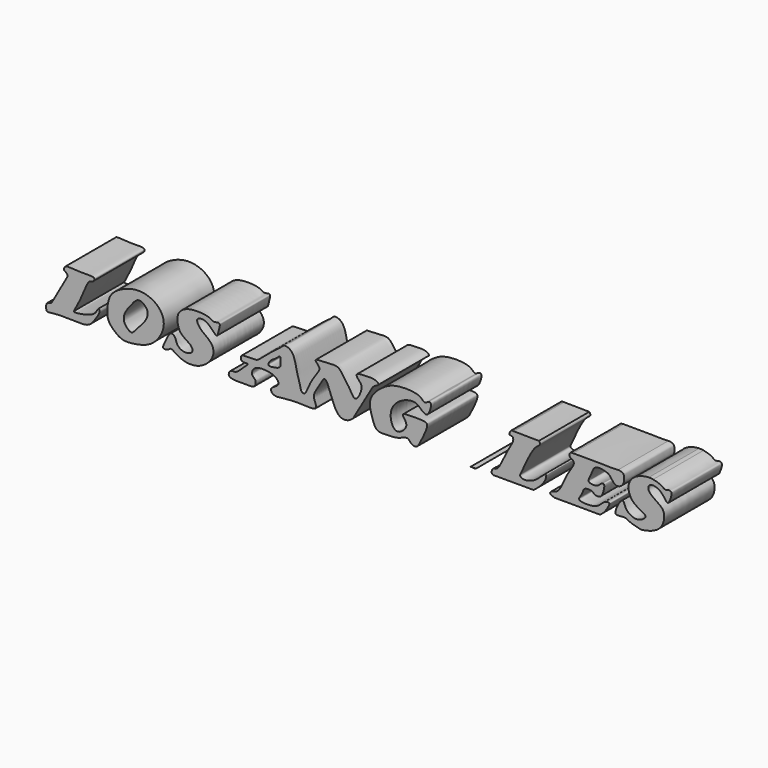
from build123d import *

# Parameters (mm, degrees)
F1_DEPTH = 6.35


# Not quite as in the source:
# - ends of sketch curves that miss each other by under 0.0002 mm in the source are joined


with BuildPart() as f1:
    # F0 (on Front) → F1 (new body)
    with BuildSketch(Plane.XZ):
        with BuildLine():
            add(Edge.make_bspline(
                [(34.4768658758, 14.4737295806), (34.5112801396, 14.4727928271), (34.5458290764, 14.4718709509), (34.5805155984, 14.4709650204)],
                knots=[0.1339558737, 0.1339558737, 0.1339558737, 0.1339558737, 0.1355001097, 0.1355001097, 0.1355001097, 0.1355001097], degree=3))
            add(Edge.make_bspline(
                [(32.5323011747, 9.9067027403), (32.4541670227, 9.9458683585), (32.2751985665, 10.0359966209), (32.4559030704, 10.5729919592), (33.0380168387, 10.4343131271), (33.7711108369, 12.3849964852), (34.5440521378, 13.3995929427), (34.5514155398, 14.0179867081), (34.0324043055, 13.9529814102), (34.2602520135, 14.4479078637), (34.3605137665, 14.4750049981), (34.4768658758, 14.4737295806)],
                knots=[0, 0, 0, 0, 0.027275365, 0.0627849405, 0.0982497275, 0.1752234358, 0.2407914191, 0.2763534131, 0.3071745918, 0.3406755244, 0.3657990569, 0.3657990569, 0.3657990569, 0.3657990569], degree=3))
            add(Edge.make_bspline(
                [(36.5833330066, 9.9053008405), (35.8773893638, 9.9053517321), (34.5279863227, 9.9056091902), (33.1766399411, 9.906295485), (32.5323011747, 9.9067027403)],
                knots=[0.3335392416, 0.3335392416, 0.3335392416, 0.3335392416, 0.4992416228, 0.6501179017, 0.6501179017, 0.6501179017, 0.6501179017], degree=3))
            add(Edge.make_bspline(
                [(37.1199468026, 14.44261028), (37.1519343343, 14.416070329), (37.3677863804, 14.1054250224), (36.4958158296, 13.8301801861), (35.3957687547, 11.0844620344), (35.1546346981, 10.7403969365), (35.5033492144, 10.4136849439), (36.7420555717, 10.676933918), (37.4847481052, 11.5347630695), (37.9200843344, 11.7919258834), (37.7947972791, 11.0937092918), (37.2140296799, 10.4098376288), (36.7884678122, 10.0690914927), (36.5833330066, 9.9053008405)],
                knots=[0.4725030515, 0.4725030515, 0.4725030515, 0.4725030515, 0.5005206768, 0.547700524, 0.6430035296, 0.6760154724, 0.7072056983, 0.7676589039, 0.8284944996, 0.8577824993, 0.8962629012, 0.950243921, 1, 1, 1, 1], degree=3))
            add(Edge.make_bspline(
                [(37.063521727, 14.4425428083), (37.0823137295, 14.442561699), (37.1011223418, 14.4425842176), (37.1199468026, 14.44261028)],
                knots=[0.1692239715, 0.1692239715, 0.1692239715, 0.1692239715, 0.1699378637, 0.1699378637, 0.1699378637, 0.1699378637], degree=3))
            add(Edge.make_bspline(
                [(34.5805155984, 14.4709650204), (35.1314661418, 14.453172138), (36.817595789, 14.4071514338), (37.063521727, 14.4425428083)],
                knots=[0.3721506797, 0.3721506797, 0.3721506797, 0.3721506797, 0.459357375, 0.459357375, 0.459357375, 0.459357375], degree=3))
        make_face()
    extrude(amount=F1_DEPTH)


with BuildPart() as f1b:
    # F0 (on Front) → F1, piece 2 (new body)
    with BuildSketch(Plane.XZ):
        with BuildLine():
            add(Edge.make_bspline(
                [(30.7684035639, 9.9080042533), (30.5910978256, 9.9081525219), (30.4137778692, 9.9083056652), (30.2364464497, 9.9084633249)],
                knots=[0.7877417533, 0.7877417533, 0.7877417533, 0.7877417533, 0.8292299046, 0.8292299046, 0.8292299046, 0.8292299046], degree=3))
            add(Edge.make_bspline(
                [(30.2364464497, 9.9084633249), (30.2480434796, 9.9076282603), (30.4475423088, 9.8919898642), (30.645100962, 9.8532213871), (30.7667153143, 9.907231483), (30.7684035639, 9.9080042533)],
                knots=[0.026563246, 0.026563246, 0.026563246, 0.026563246, 0.0277484383, 0.0470040149, 0.0472770858, 0.0472770858, 0.0472770858, 0.0472770858], degree=3))
        make_face()
    extrude(amount=F1_DEPTH)


with BuildPart() as f1c:
    # F0 (on Front) → F1, piece 3 (new body)
    with BuildSketch(Plane.XZ):
        with BuildLine():
            add(Edge.make_bspline(
                [(38.718625811, 9.9052852467), (38.5135813539, 9.965903255), (38.1634283773, 10.0694614859), (38.3624359939, 10.4577232253), (39.1171957291, 10.4145474294), (39.6140354439, 11.7570882036), (40.264894038, 12.9054629976), (40.6644877345, 13.432394025), (40.6342538489, 13.8855215631), (40.0886665403, 14.024998654), (40.2583159891, 14.4507891646), (40.3653461826, 14.4606033405), (40.5612274768, 14.467808711)],
                knots=[0, 0, 0, 0, 0.0234493646, 0.0400679945, 0.0658311953, 0.1038715824, 0.1427742296, 0.1688455969, 0.1884932671, 0.2104317591, 0.2283583247, 0.2468497136, 0.2468497136, 0.2468497136, 0.2468497136], degree=3))
            add(Edge.make_bspline(
                [(40.8433932409, 9.9057387335), (40.1351970665, 9.905587584), (39.4270009049, 9.9054527643), (38.718625811, 9.9052852467)],
                knots=[0, 0, 0, 0, 0.1663998621, 0.1663998621, 0.1663998621, 0.1663998621], degree=3))
            add(Edge.make_bspline(
                [(43.2678567779, 9.8901794928), (42.4617746641, 9.9157399972), (41.6392296575, 9.9329845193), (40.8433932409, 9.9057387335)],
                knots=[0.8753656822, 0.8753656822, 0.8753656822, 0.8753656822, 0.9071716793, 0.9071716793, 0.9071716793, 0.9071716793], degree=3))
            add(Edge.make_bspline(
                [(45.1012092872, 14.4622358719), (45.4844363537, 14.4274675017), (45.7750792463, 14.3040325549), (45.7165046627, 13.1471962694), (44.7314215276, 12.8484351058), (44.3446618894, 13.7318670905), (43.779898461, 13.9552776294), (42.6721876007, 14.143056728), (42.4200388298, 13.1817012223), (42.1375735513, 12.7160040765), (42.0934433991, 12.3265459652), (43.0723981196, 12.2605262747), (43.3340512659, 12.7193371486), (43.7764141603, 12.8149416944), (43.662126014, 12.1247922037), (43.4210997106, 11.3922556923), (42.6914128218, 11.455909825), (42.5215425357, 11.7876309832), (41.5794702071, 11.8011837957), (41.5631473809, 11.1619219007), (40.9386497254, 10.5104977654), (41.7920834613, 10.3487349178), (43.0985475186, 10.4282046124), (43.5927155966, 11.1933341463), (44.3976497916, 11.3538748898), (43.9912126895, 10.6478167398), (43.6448087091, 10.1523723502), (43.3841416805, 9.9713765802), (43.2678567779, 9.8901794928)],
                knots=[0.3170026618, 0.3170026618, 0.3170026618, 0.3170026618, 0.3434489893, 0.3749791608, 0.4034215732, 0.4328717168, 0.4589348824, 0.4907763547, 0.5210849698, 0.5459241096, 0.5625973731, 0.5919434389, 0.6158108763, 0.6328153746, 0.657443103, 0.6857445259, 0.7103256391, 0.729915535, 0.7580183435, 0.7829258001, 0.809539198, 0.8345757029, 0.8722584856, 0.9036550327, 0.926657814, 0.9511783368, 0.9782105166, 1, 1, 1, 1], degree=3))
            add(Edge.make_bspline(
                [(40.5612274768, 14.467808711), (41.4373321776, 14.4749541476), (43.4065275967, 14.4832914551), (44.404762779, 14.4102661712), (45.1012092872, 14.4622358719)],
                knots=[0.213383647, 0.213383647, 0.213383647, 0.213383647, 0.2482603597, 0.2988779642, 0.2988779642, 0.2988779642, 0.2988779642], degree=3))
        make_face()
    extrude(amount=F1_DEPTH)


with BuildPart() as f1d:
    # F0 (on Front) → F1, piece 4 (new body)
    with BuildSketch(Plane.XZ):
        with BuildLine():
            add(Edge.make_bspline(
                [(48.2063107618, 14.8080410421), (48.361353415, 14.8025450615), (48.5065364369, 14.7871576478), (48.6413690998, 14.7643067953)],
                knots=[0.366400242, 0.366400242, 0.366400242, 0.366400242, 0.3777635297, 0.3777635297, 0.3777635297, 0.3777635297], degree=3))
            add(Edge.make_bspline(
                [(47.4133412883, 9.9057387335), (46.9725338397, 10.0134268872), (46.2515458614, 10.1895948628), (45.850088848, 10.5125088591), (45.138855998, 10.383096561), (44.6552953768, 10.4479064453), (45.2207468206, 11.7372843188), (45.6917339954, 11.9887531473), (45.7921261937, 11.2608218345), (46.5757989122, 10.6369990891), (47.3861596047, 10.7140682616), (48.0851201046, 11.2394276569), (47.3483966756, 11.6465310313), (46.4460471609, 12.0954145822), (45.9472697626, 13.4041358945), (46.7122823199, 14.561768142), (47.8559378649, 14.7943353068), (48.2063107193, 14.8080410436)],
                knots=[0, 0, 0, 0, 0.077437218, 0.1266613719, 0.1855901369, 0.2238421303, 0.3027768951, 0.345087592, 0.3979643199, 0.4667316111, 0.5304178838, 0.5855747405, 0.6398989755, 0.7123026851, 0.7903598777, 0.8691903302, 0.9533376764, 0.9533376764, 0.9533376764, 0.9533376764], degree=3))
            add(Edge.make_bspline(
                [(48.6413690998, 14.7643067953), (49.001027409, 14.7033534715), (49.5110446895, 14.4999664824), (49.8485973579, 14.1905299076), (50.1520312715, 14.3484072118), (50.6416228519, 14.3040310738), (50.3264757069, 13.4051786644), (50.0922791452, 12.9863703016), (49.6665779866, 13.6956729791), (49.1647749556, 14.1531007966), (48.2986025006, 14.3401157398), (47.9873927024, 13.6104758419), (49.0101373653, 12.9095010149), (49.8719114445, 12.3722330399), (49.6878282098, 10.5866768403), (48.4221076097, 10.0353934607), (47.4133412883, 9.9057387335)],
                knots=[0.3777635297, 0.3777635297, 0.3777635297, 0.3777635297, 0.4080744409, 0.4318138392, 0.4518618025, 0.472205762, 0.5054119396, 0.5260348343, 0.5547091476, 0.5863153403, 0.6174273922, 0.6432110306, 0.6815114437, 0.7172127576, 0.7596173353, 0.8144781544, 0.8144781544, 0.8144781544, 0.8144781544], degree=3))
        make_face()
    extrude(amount=F1_DEPTH)


with BuildPart() as f1e:
    # F0 (on Front) → F1, piece 5 (new body)
    with BuildSketch(Plane.XZ):
        with BuildLine():
            add(Edge.make_bspline(
                [(-9.7831104874, 10.7108312697), (-9.5950454946, 11.093317591), (-9.2860023376, 11.7217945983), (-9.0581878575, 12.0865172653), (-8.5637830889, 13.3512127314), (-8.2448274482, 13.9212845659), (-7.8305533182, 13.9063295694), (-7.6446188222, 14.3012483336), (-8.0264709842, 14.4262921763), (-8.8381735222, 14.3667908405), (-10.1439046456, 14.4448887029), (-10.6660898244, 14.4953689384), (-10.8636029298, 14.0294127442), (-10.5848318503, 13.9224699449), (-10.3791844836, 13.6672874639), (-10.4643739569, 13.5103759365), (-10.5048306286, 13.4358583018)],
                knots=[0.0001566694, 0.0001566694, 0.0001566694, 0.0001566694, 0.1031082956, 0.1694222377, 0.2827346198, 0.359654875, 0.417114896, 0.4710627289, 0.5224264412, 0.6128031166, 0.7262449494, 0.793312149, 0.8512485611, 0.8997805232, 0.9524055698, 1, 1, 1, 1], degree=3))
            add(Edge.make_bspline(
                [(-10.5048306286, 13.4358583018), (-11.111802213, 12.355849674), (-11.9073362504, 10.9403243905), (-12.0884096109, 10.6229939383), (-12.5134287105, 10.6403297729), (-12.6107940514, 10.2661819977), (-12.5751779421, 9.6841727582), (-11.8093591696, 9.9133287705), (-9.4218227173, 9.8703548386), (-8.8075229584, 9.8202820579), (-8.0408529888, 10.0242220176), (-7.5418327302, 10.8534472885), (-7.099782311, 11.474480533), (-7.3315011816, 11.8740905081), (-7.5528421638, 11.1609376867), (-8.3507527089, 10.8513853859), (-9.1455907434, 10.6458267455), (-9.7541621378, 10.6050908929), (-9.7812796189, 10.6909704053), (-9.7831104874, 10.7108312697)],
                knots=[0, 0, 0, 0, 0.1223676782, 0.1603825543, 0.201389393, 0.2434286791, 0.2904717262, 0.3475918385, 0.4588206991, 0.5171187103, 0.5761489951, 0.6470845322, 0.7084840664, 0.7415904522, 0.7929674686, 0.8591802712, 0.9271226938, 0.9792659839, 0.9934126503, 0.9934126503, 0.9934126503, 0.9934126503], degree=3))
        make_face()
    extrude(amount=F1_DEPTH)


with BuildPart() as f1f:
    # F0 (on Front) → F1, piece 6 (new body)
    with BuildSketch(Plane.XZ):
        with BuildLine():
            add(Edge.make_bspline(
                [(-5.9119630605, 10.4841180146), (-6.1036939558, 10.6784201151), (-6.4221233493, 11.0480734957), (-6.4396892173, 12.2965647029), (-6.1372585796, 13.5029134325), (-4.8744149654, 14.3512139958), (-3.2895880396, 14.7940159404), (-1.6139891323, 14.3540043474), (-0.6206388277, 13.1356209217), (-0.7539352118, 11.6498263262), (-1.9305291345, 10.1347618448), (-3.6588662383, 9.7564012308), (-5.0124344733, 9.6391651222), (-5.6728543676, 10.241802757), (-5.9119630605, 10.4841180146)],
                knots=[0, 0, 0, 0, 0.060955485, 0.1382878927, 0.2165469674, 0.3017686672, 0.3928667622, 0.484409508, 0.569462374, 0.6528699079, 0.7486580595, 0.8426240387, 0.923982067, 1, 1, 1, 1], degree=3))
        make_face()
        with BuildLine():
            add(Edge.make_bspline(
                [(-4.7054300085, 11.4048924297), (-4.8221480388, 11.7486095831), (-4.5870889049, 12.4341394937), (-4.034172335, 13.1202884214), (-3.4565337255, 13.8525328756), (-2.8552184683, 13.799515972), (-2.1060569123, 13.0199090142), (-2.7246014826, 11.8831877525), (-3.5814458227, 11.0918676538), (-3.9864616129, 10.481888247), (-4.5895573421, 11.0636647467), (-4.7054300085, 11.4048924297)],
                knots=[0, 0, 0, 0, 0.1182200316, 0.2324666919, 0.3420396722, 0.4265101549, 0.5379656341, 0.6653597964, 0.7970240743, 0.882636211, 1, 1, 1, 1], degree=3))
        make_face(mode=Mode.SUBTRACT)
    extrude(amount=F1_DEPTH)


with BuildPart() as f1g:
    # F0 (on Front) → F1, piece 7 (new body)
    with BuildSketch(Plane.XZ):
        with BuildLine():
            add(Edge.make_bspline(
                [(0.4699597484, 10.293613188), (0.7574562614, 10.1044257186), (1.5535933325, 9.7146434792), (3.1796142044, 9.8733788995), (4.3978340553, 11.1582283833), (4.2705109721, 12.3315945233), (3.3089292998, 12.9935823276), (2.8901135221, 13.3333877966), (2.4471656096, 14.0984586845), (3.2986315081, 14.3021584732), (3.9174967161, 13.8696913343), (4.3026192063, 13.437664805), (4.6870111816, 13.0683357103), (4.8053063064, 13.6924092946), (5.0764080208, 14.5865806517), (4.3122850597, 14.2504657489), (3.9448177363, 14.632720012), (2.7844636904, 14.7893824552), (1.4650108956, 14.6733905536), (0.5269906015, 13.9096755955), (0.7253991308, 12.5212727386), (1.2861776079, 11.9489440846), (2.0271881956, 11.5905769585), (2.3432271281, 10.8988021273), (1.3409244438, 10.5654772566), (0.5604125909, 11.0426175409), (0.4756326632, 11.7805735833), (-0.1051893607, 12.0899215929), (-0.5038787585, 11.0776417547), (-0.9952269424, 10.2290005562), (-0.2441765396, 10.3439314268), (-0.0060648378, 10.657680197), (0.2754833077, 10.4215886729), (0.4699597484, 10.293613188)],
                knots=[0, 0, 0, 0, 0.0396357344, 0.0856226469, 0.1322708745, 0.1693276591, 0.2074249623, 0.2359953421, 0.2654082911, 0.293880305, 0.3257059138, 0.3547905916, 0.376288161, 0.4025607577, 0.43328263, 0.4594539682, 0.4849642214, 0.5239154784, 0.5664910827, 0.6041773707, 0.6450577979, 0.6776350108, 0.7108406138, 0.7376026449, 0.7706954952, 0.8042929622, 0.8349040744, 0.8583051318, 0.8952880604, 0.9266949197, 0.952038606, 0.9731884868, 1, 1, 1, 1], degree=3))
        make_face()
    extrude(amount=F1_DEPTH)


with BuildPart() as f1h:
    # F0 (on Front) → F1, piece 8 (new body)
    with BuildSketch(Plane.XZ):
        with BuildLine():
            add(Edge.make_bspline(
                [(7.6456540264, 9.8491003737), (7.172639711, 9.8554229723), (6.259624141, 9.7865500549), (5.7190906846, 10.071101), (5.9924663699, 10.6823534344), (6.5537511643, 10.4765331621), (7.2047294953, 11.1755496685), (7.5667605092, 11.4779824792), (7.9066843756, 11.8250468776), (7.0186346363, 11.604523958), (7.040893338, 12.3448676011), (7.4922693373, 12.309502418), (8.4807284038, 12.3678997982), (8.7010081948, 12.3461110143), (9.3967767527, 12.9065855876), (10.1576355547, 13.6247084399), (11.1489418593, 14.2851706849), (11.417995936, 14.6467502458), (12.4583376493, 14.3636188169), (12.6963580429, 12.4169727285), (13.0372101158, 11.6617540198), (13.0851847517, 11.0309858411), (13.6019147765, 10.7985246156), (13.9967375658, 12.2920217667), (15.1369697655, 13.5539269668), (14.8814705397, 13.8940783397), (14.4239215289, 14.3717367112), (15.0977998222, 14.3866455239), (16.0413010533, 14.4552104452), (16.8727168633, 14.4979047377), (17.3525593946, 13.8476048917), (18.0165849701, 12.9701026409), (18.5811614361, 11.7721333957), (19.2207462725, 12.9522397382), (19.2638914114, 13.6490234791), (18.8455007492, 13.9891976549), (18.588896749, 14.5282916861), (19.6988470811, 14.490407516), (20.4580576617, 14.5962461503), (21.1644147461, 14.1746897005), (20.4430316602, 13.9553355332), (20.0930454297, 13.3284076422), (18.7451627346, 11.0894280694), (18.2930307549, 10.0441589129), (16.8579397405, 9.748290198), (16.1523122997, 11.6141512934), (15.5618774123, 13.3143357807), (15.040461801, 12.2049152511), (14.2772147346, 11.1928263234), (14.5588162406, 10.527406533), (14.812892286, 9.786978836), (13.0222902335, 9.9589454349), (11.6151641478, 9.8955046274), (10.3335233563, 9.6527478299), (9.941412308, 10.3189324826), (10.514179565, 10.5918313811), (11.0053077027, 10.9696000459), (10.5569113057, 11.5153173618), (9.9530299263, 11.7270513324), (8.6607491478, 11.8383342962), (8.1514484274, 11.3010009662), (8.1807418805, 10.7487943173), (8.5963356088, 10.6183372547), (8.5410134687, 9.7833824683), (8.0004093513, 9.844358497), (7.6456540264, 9.8491003737)],
                knots=[0, 0, 0, 0, 0.0215577001, 0.0337604743, 0.0459190053, 0.0584187554, 0.0753616434, 0.0888770349, 0.097505692, 0.1111801792, 0.1232638815, 0.1345648492, 0.1524600366, 0.1610045127, 0.1770706853, 0.1965838392, 0.2159702086, 0.227196574, 0.2432884068, 0.2679324264, 0.2849838566, 0.2985100361, 0.3084070146, 0.3297924148, 0.3528793823, 0.3634246291, 0.3756274033, 0.3873641324, 0.405839698, 0.4216085382, 0.4368933338, 0.4569169782, 0.4740484727, 0.4914744267, 0.5065536172, 0.5195667128, 0.5304166783, 0.5472040266, 0.5645129673, 0.5772899196, 0.5894926835, 0.6053021434, 0.6343970632, 0.6538417047, 0.6720583086, 0.6972366948, 0.7179597691, 0.7337692305, 0.7542701457, 0.769126814, 0.7815854352, 0.8031643846, 0.8263439232, 0.8458892704, 0.8584432563, 0.8717032168, 0.8846676557, 0.8977764416, 0.9126896801, 0.9327563324, 0.9473113661, 0.959349498, 0.9701574856, 0.9838319716, 1, 1, 1, 1], degree=3))
        make_face()
        with BuildLine():
            add(Edge.make_bspline(
                [(9.8364632577, 12.2939161956), (9.9164419046, 12.1881244581), (10.5159028251, 12.310111925), (10.7349759981, 12.3254492899), (11.1394706358, 12.5656936343), (10.9995109067, 12.9508786935), (11.1203429279, 13.6669102003), (10.5317641074, 13.0232618014), (10.105845251, 12.9142985898), (9.760824068, 12.3939679171), (9.8364632577, 12.2939161956)],
                knots=[0, 0, 0, 0, 0.1449151087, 0.2433057124, 0.3527226254, 0.4695569739, 0.5909561564, 0.7253631517, 0.8629476515, 1, 1, 1, 1], degree=3))
        make_face(mode=Mode.SUBTRACT)
    extrude(amount=F1_DEPTH)


with BuildPart() as f1i:
    # F0 (on Front) → F1, piece 9 (new body)
    with BuildSketch(Plane.XZ):
        with BuildLine():
            add(Edge.make_bspline(
                [(20.7905098796, 10.10310743), (20.5279205103, 10.2979696507), (20.2256126174, 11.2666396102), (19.8198801888, 12.7680640905), (21.6403577385, 14.4160634557), (23.1869896409, 14.7904560933), (25.1767876948, 14.6798095987), (25.571814028, 13.9269801395), (25.9738818375, 14.3674982341), (26.3482946224, 14.2322998066), (26.0913923473, 13.3872559427), (25.8046048662, 12.963637884), (25.2063273408, 13.3399602419), (24.6857297878, 13.9990785442), (23.001477011, 13.5715193078), (22.0409224154, 12.3535806731), (22.215976026, 11.000870013), (22.9094988619, 10.4089265018), (23.9056278612, 11.2773723548), (23.6418970118, 11.9243201061), (23.159871936, 12.4514128875), (24.4007174376, 12.4451477561), (25.5094652686, 12.4819903464), (26.0618243133, 12.2368443617), (25.1989470736, 10.5365646211), (24.7932047428, 9.742077402), (24.1672332536, 9.9912239102), (23.9084029604, 10.550880445), (22.9117408572, 9.9725380656), (21.6847681584, 9.996650065), (21.0104399912, 9.9399017753), (20.7905098796, 10.10310743)],
                knots=[0, 0, 0, 0, 0.0399593861, 0.0834531513, 0.1362384071, 0.1833651016, 0.2323822019, 0.2600106577, 0.2834748319, 0.3011533046, 0.3334989397, 0.3569956731, 0.3840897479, 0.4157416032, 0.4602483858, 0.5041707192, 0.5442810087, 0.5740763692, 0.610680203, 0.6396110308, 0.6630752051, 0.6977355119, 0.7377475661, 0.7593783838, 0.8071937788, 0.8401088896, 0.8655814535, 0.8902807824, 0.9254165428, 0.9665322619, 1, 1, 1, 1], degree=3))
        make_face()
    extrude(amount=F1_DEPTH)


solid = Compound([f1.part, f1b.part, f1c.part, f1d.part, f1e.part, f1f.part, f1g.part, f1h.part, f1i.part])
